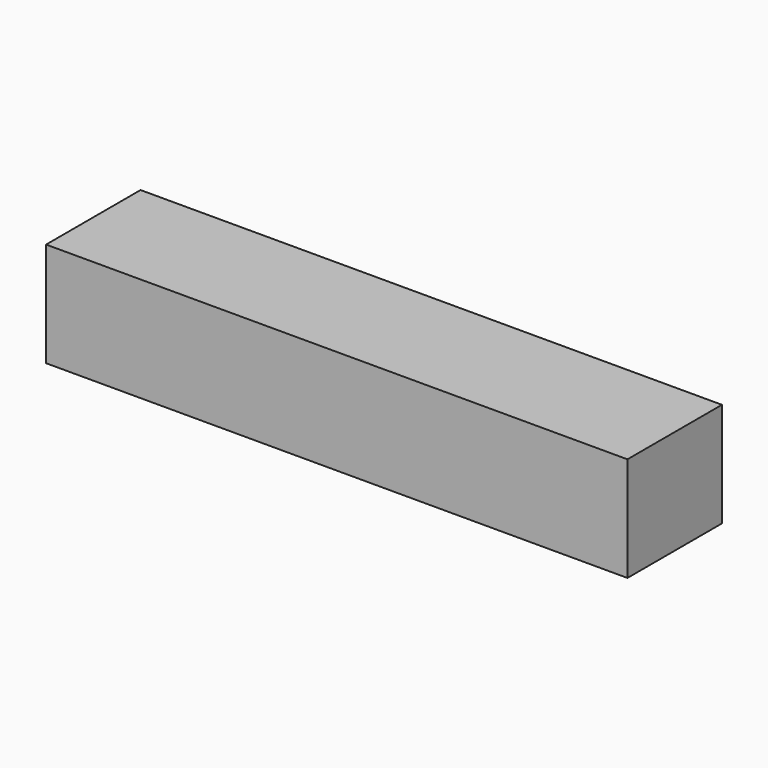
from build123d import *

# Parameters (mm, degrees)
F0_W     = 128
F0_H     = 26
F1_DEPTH = 4
F3_DEPTH = 15
F4_W     = 128
F4_H     = 26
F5_DEPTH = 4


# Not quite as in the source:
# - a feature names something its author has since deleted; it is built from what else it names


with BuildPart() as f1:
    # F0 (on Top) → F1 (new body)
    with BuildSketch(Plane.XY):
        with Locations((-64, -13)):
            Rectangle(F0_W, F0_H)
    extrude(amount=F1_DEPTH)

    # F2 (on face) → F3 (join)
    with BuildSketch(Plane.XY.offset(4)):
        Polygon((-88.4999999069, 0), (-103.4999999069, 0), (-103.4999999069, -14.9287388836), (-118.4999999069, -14.9287388836), (-118.4999999069, 0), (-128, 0), (-128, -26), (0, -26), (0, 0), (-13.5, 0), (-13.5, -15.0637076219), (-28.5, -15.0637076219), (-28.5, 0), (-43.4999999069, 0), (-43.4999999069, -15), (-58.4999999069, -15), (-58.4999999069, 0), (-73.4999999069, 0), (-73.4999999069, -15.0510713975), (-88.4999999069, -15.0510713975), align=None)
    extrude(amount=F3_DEPTH)

    # F4 (on face) → F5 (join)
    with BuildSketch(Plane.XY.offset(19)):
        with Locations((-64, -13)):
            Rectangle(F4_W, F4_H)
    extrude(amount=F5_DEPTH)


solid = f1.part
